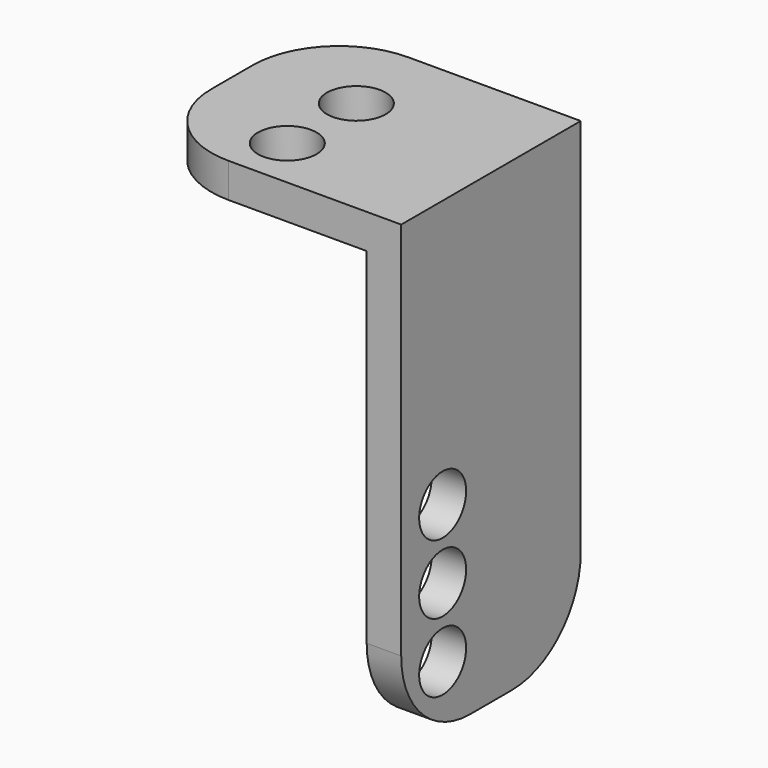
from build123d import *

# Parameters (mm, degrees)
F0_W     = 2
F0_H     = 20
F0_W_2   = 13
F1_DEPTH = 2
F2_D     = 3.4
F3_DEPTH = 25
F5_D     = 3.4
F6_DEPTH = 7
F7_R     = 5


with BuildPart() as f1:
    # F0 (on Top) → F1 (new body)
    with BuildSketch(Plane.XY):
        with Locations((6.5, 0)):
            Rectangle(F0_W, F0_H)
        with Locations((-1, 0)):
            Rectangle(F0_W_2, F0_H)
    extrude(amount=F1_DEPTH)

    # F2 (through all)
    with Locations(Plane(origin=(0, 0, 0), x_dir=(1, 0, 0), z_dir=(0, 0, -1))):
        with Locations((-1.5, -5), (-1.5, 0), (-1.5, 5)):
            Hole(F2_D / 2)

    # F0 (on Top) → F3 (join)
    with BuildSketch(Plane.XY):
        with Locations((6.5, 0)):
            Rectangle(F0_W, F0_H)
    extrude(amount=-F3_DEPTH)

    # F5 (through all)
    with Locations(Plane(origin=(5.5, 0, 0), x_dir=(0, -1, 0), z_dir=(-1, 0, 0))):
        with Locations((0, -17.5), (0, -13.5), (0, -21.5)):
            Hole(F5_D / 2)

    # F6 (cut): a face of the model
    f6_faces = [f1.faces().sort_by_distance(p)[0] for p in [
        (-7.1911310958, -10, 1),
    ]]
    extrude(f6_faces, amount=-F6_DEPTH, mode=Mode.SUBTRACT)

    # F7
    f7_edges = [f1.edges().sort_by_distance(p)[0] for p in [
        (-7.5, -3, 1),
        (-7.5, 10, 1),
        (6.5, 10, -25),
        (6.5, -3, -25),
    ]]
    fillet(f7_edges, radius=F7_R)


solid = f1.part
